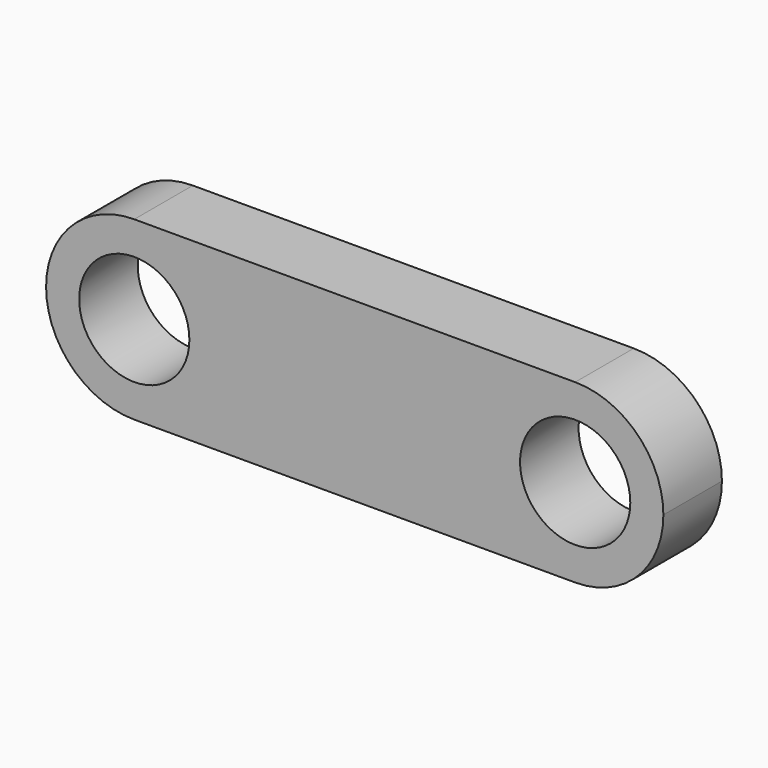
from build123d import *

# Parameters (mm, degrees)
F1_DEPTH = 25.2984


with BuildPart() as f1:
    # F0 (on Front) → F1 (new body)
    with BuildSketch(Plane.XZ):
        with BuildLine():
            ThreePointArc((76.2, -30.48), (45.72, 0), (76.2, 30.48))
            Line((76.2, 30.48), (-76.2, 30.48))
            ThreePointArc((-76.2, 30.48), (-54.6473853094, 21.5526146906), (-45.72, 0))
            ThreePointArc((-45.72, 0), (-54.6473853094, -21.5526146906), (-76.2, -30.48))
            Line((-76.2, -30.48), (76.2, -30.48))
        make_face()
        with BuildLine():
            ThreePointArc((106.68, 0), (97.7526146906, 21.5526146906), (76.2, 30.48))
            Line((76.2, 30.48), (76.2, 19.05))
            ThreePointArc((76.2, 19.05), (89.6703841816, 13.4703841816), (95.25, 0))
            ThreePointArc((95.25, 0), (89.6703841816, -13.4703841816), (76.2, -19.05))
            Line((76.2, -19.05), (76.2, -30.48))
            ThreePointArc((76.2, -30.48), (97.7526146906, -21.5526146906), (106.68, 0))
        make_face()
        with BuildLine():
            Line((76.2, 19.05), (76.2, 30.48))
            ThreePointArc((76.2, 30.48), (45.72, 0), (76.2, -30.48))
            Line((76.2, -30.48), (76.2, -19.05))
            ThreePointArc((76.2, -19.05), (57.15, 0), (76.2, 19.05))
        make_face()
        with BuildLine():
            ThreePointArc((-45.72, 0), (-54.6473853094, 21.5526146906), (-76.2, 30.48))
            Line((-76.2, 30.48), (-76.2, 19.05))
            ThreePointArc((-76.2, 19.05), (-62.7296158184, 13.4703841816), (-57.15, 0))
            ThreePointArc((-57.15, 0), (-62.7296158184, -13.4703841816), (-76.2, -19.05))
            Line((-76.2, -19.05), (-76.2, -30.48))
            ThreePointArc((-76.2, -30.48), (-54.6473853094, -21.5526146906), (-45.72, 0))
        make_face()
        with BuildLine():
            Line((-76.2, 19.05), (-76.2, 30.48))
            ThreePointArc((-76.2, 30.48), (-106.68, 0), (-76.2, -30.48))
            Line((-76.2, -30.48), (-76.2, -19.05))
            ThreePointArc((-76.2, -19.05), (-95.25, 0), (-76.2, 19.05))
        make_face()
    extrude(amount=F1_DEPTH)


solid = f1.part
